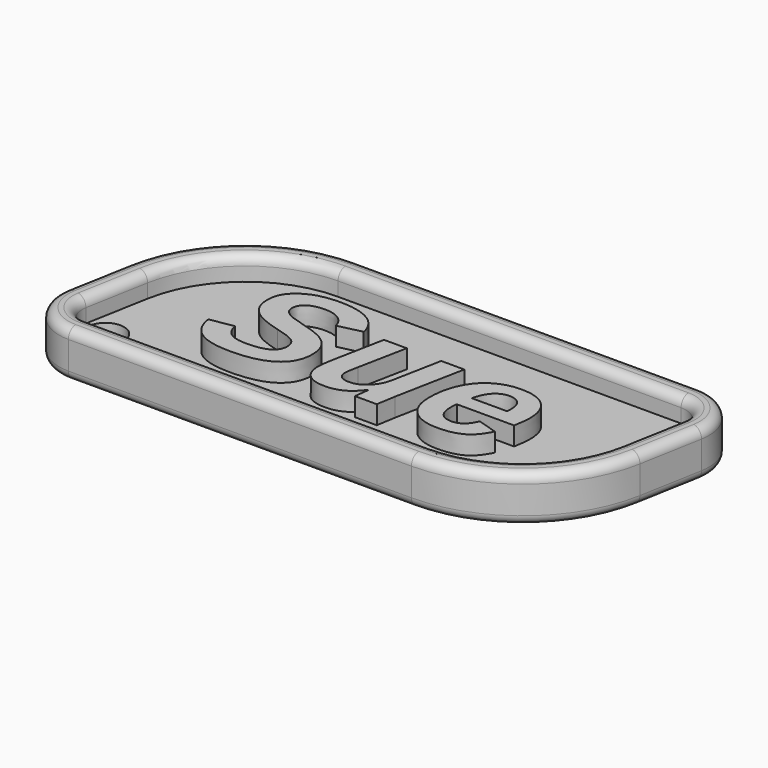
from build123d import *

# Parameters (mm, degrees)
F1_DEPTH     = 5
F0_R         = 2
F2_DEPTH     = 2.5
F3_TEXT_SIZE = 18.0555555556
F4_DEPTH     = 2
F5_R         = 1


# Not quite as in the source:
# - Text() gives the source's letters only with a copy of the font that has no kerning and outlines rounded to 1/6400 em; it was checked with that copy


with BuildPart() as f1:
    # F0 (on Top) → F1 (new body)
    with BuildSketch(Plane.XY):
        with BuildLine():
            ThreePointArc((28.937473683, 6.6120529013), (27.8535983251, 10.7062645326), (24.0169503419, 12.5))
            Line((24.0169503419, 12.5), (-12.953140312, 12.5))
            ThreePointArc((-12.953140312, 12.5), (-22.5719339099, 9.0099439495), (-27.7147103351, 0.163841296))
            Line((-27.7147103351, 0.163841296), (-28.937473683, -6.6120529013))
            ThreePointArc((-28.937473683, -6.6120529013), (-27.8535983251, -10.7062645326), (-24.0169503419, -12.5))
            Line((-24.0169503419, -12.5), (12.953140312, -12.5))
            ThreePointArc((12.953140312, -12.5), (22.5719339099, -9.0099439495), (27.7147103351, -0.163841296))
            Line((27.7147103351, -0.163841296), (28.937473683, 6.6120529013))
        make_face()
        with BuildLine():
            ThreePointArc((24.0169503419, 10), (25.9352743335, 9.1031322663), (26.4772120124, 7.0560264507))
            Line((26.4772120124, 7.0560264507), (25.2544486646, 0.2801322533))
            ThreePointArc((25.2544486646, 0.2801322533), (20.9688016436, -7.0916199579), (12.953140312, -10))
            Line((12.953140312, -10), (-24.0169503419, -10))
            ThreePointArc((-24.0169503419, -10), (-25.9352743335, -9.1031322663), (-26.4772120124, -7.0560264507))
            Line((-26.4772120124, -7.0560264507), (-25.2544486646, -0.2801322533))
            ThreePointArc((-25.2544486646, -0.2801322533), (-20.9688016436, 7.0916199579), (-12.953140312, 10))
            Line((-12.953140312, 10), (24.0169503419, 10))
        make_face(mode=Mode.SUBTRACT)
    extrude(amount=F1_DEPTH)

    # F0 (on Top) → F2 (join)
    with BuildSketch(Plane.XY):
        with BuildLine():
            Line((25.2544486646, 0.2801322533), (26.4772120124, 7.0560264507))
            ThreePointArc((26.4772120124, 7.0560264507), (25.9352743335, 9.1031322663), (24.0169503419, 10))
            Line((24.0169503419, 10), (-12.953140312, 10))
            ThreePointArc((-12.953140312, 10), (-20.9688016436, 7.0916199579), (-25.2544486646, -0.2801322533))
            Line((-25.2544486646, -0.2801322533), (-26.4772120124, -7.0560264507))
            ThreePointArc((-26.4772120124, -7.0560264507), (-25.9352743335, -9.1031322663), (-24.0169503419, -10))
            Line((-24.0169503419, -10), (12.953140312, -10))
            ThreePointArc((12.953140312, -10), (20.9688016436, -7.0916199579), (25.2544486646, 0.2801322533))
        make_face()
        with Locations((-24.0169503419, -7.5)):
            Circle(F0_R, mode=Mode.SUBTRACT)
    extrude(amount=F2_DEPTH)

    # F3 (on face) → F4 (join)
    with BuildSketch(Plane.XY.offset(2.5)):
        with Locations((-16.7320842616, -6.2523214242)):
            Text('Sue', F3_TEXT_SIZE, font='Arimo', font_style=FontStyle.BOLDITALIC, text_align=(TextAlign.LEFT, TextAlign.BOTTOM))
    extrude(amount=F4_DEPTH)

    # F5
    f5_edges = [f1.edges().sort_by_distance(p)[0] for p in [
        (27.853598, 10.706265, 5),
        (5.531905, 12.5, 5),
        (-22.571934, 9.009944, 5),
        (-28.326092, -3.224106, 5),
        (-27.853598, -10.706265, 5),
        (-5.531905, -12.5, 5),
        (22.571934, -9.009944, 5),
        (28.326092, 3.224106, 5),
        (-20.968802, 7.09162, 5),
        (5.531905, 10, 5),
        (25.935274, 9.103132, 5),
        (25.86583, 3.668079, 5),
        (20.968802, -7.09162, 5),
        (-5.531905, -10, 5),
        (-25.935274, -9.103132, 5),
        (-25.86583, -3.668079, 5),
        (27.853598, 10.706265, 0),
        (5.531905, 12.5, 0),
        (-22.571934, 9.009944, 0),
        (-28.326092, -3.224106, 0),
        (-27.853598, -10.706265, 0),
        (-5.531905, -12.5, 0),
        (22.571934, -9.009944, 0),
        (28.326092, 3.224106, 0),
        (-26.01695, -7.5, 0),
    ]]
    fillet(f5_edges, radius=F5_R)


solid = f1.part
